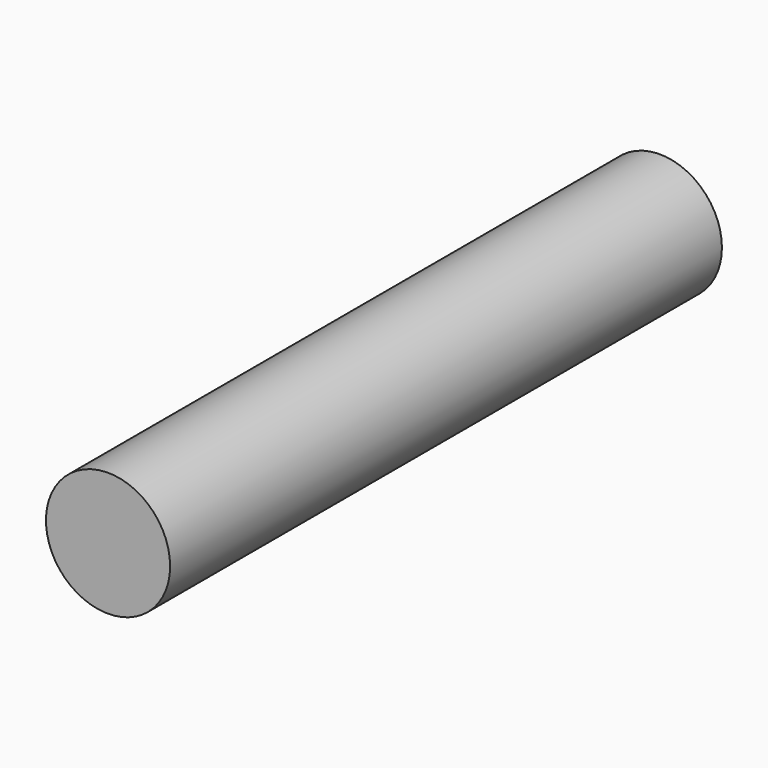
from build123d import *

# Parameters (mm, degrees)
F0_R     = 11.43
F1_DEPTH = 127


# Not quite as in the source:
# - a feature names something its author has since deleted; it is built from what else it names


with BuildPart() as f1:
    # F0 (on Front) → F1 (new body)
    with BuildSketch(Plane.XZ):
        Circle(F0_R)
    extrude(amount=F1_DEPTH)


solid = f1.part
